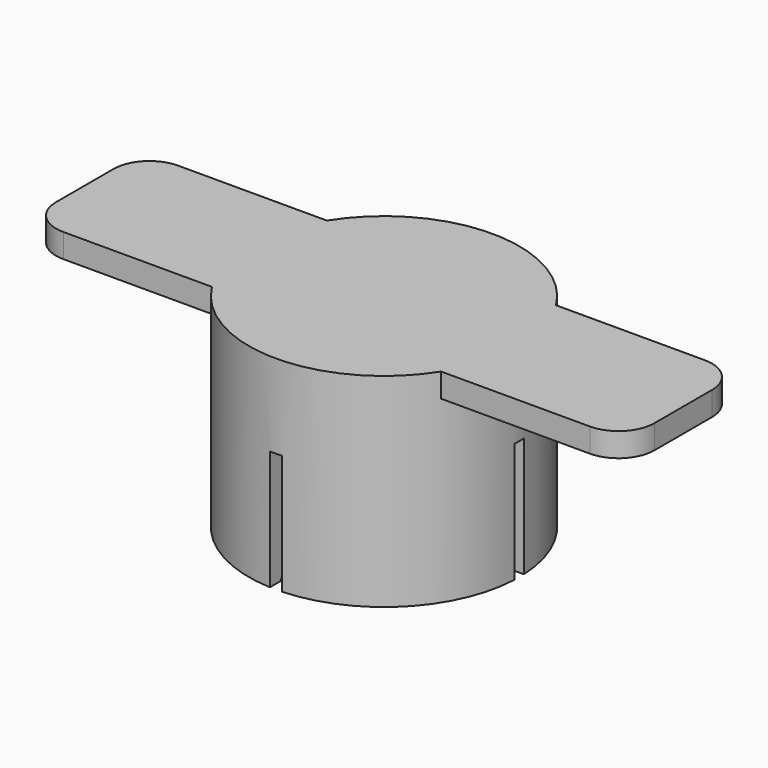
from build123d import *

# Parameters (mm, degrees)
F0_R         = 11.3
F0_R_2       = 9
F1_DEPTH     = 15
F2_R         = 11.3
F3_DEPTH     = 2
F5_START     = -5
F4_R         = 9.5
F4_R_2       = 7.1437360255
F5_DEPTH     = 3.1
F7_W         = 50
F7_H         = 12
F8_DEPTH     = 2
F9_R         = 3
F10_W        = 1
F10_H        = 12
F10_W_2      = 12
F10_H_2      = 1
F11_DEPTH    = 10
F12_SIZE     = 1.2
F13_T2_ANGLE = 179.6107254138
F13_T4_ANGLE = 179.6107254138
F13_T6_ANGLE = 179.6107254138
F13_T8_ANGLE = 179.6107254138


# Not quite as in the source:
# - a fillet or chamfer that OpenCascade refuses, or shapes differently, is made with other operations: its cross-section is extruded or revolved along the edge and cut away or added


with BuildPart() as f1:
    # F0 (on Top) → F1 (new body)
    with BuildSketch(Plane.XY):
        Circle(F0_R)
        Circle(F0_R_2, mode=Mode.SUBTRACT)
    extrude(amount=F1_DEPTH)

    # F2 (on face) → F3 (join)
    with BuildSketch(Plane.XY.offset(15)):
        Circle(F2_R)
    extrude(amount=F3_DEPTH)

    # F4 (on face) → F5 (cut)
    with BuildSketch(Plane(origin=(0, 0, 0), x_dir=(1, 0, 0), z_dir=(0, 0, -1)).offset(F5_START)):
        Circle(F4_R)
        Circle(F4_R_2, mode=Mode.SUBTRACT)
    extrude(amount=-F5_DEPTH, mode=Mode.SUBTRACT)

    # F6: fillet of radius 1.5 on 3 edges, made by hand

    # F6_s1 → F6_t2 (revolve)
    with BuildSketch(Plane.XZ):
        with BuildLine():
            ThreePointArc((9, 5), (9.3693063938, 5.5056615531), (9.5, 6.1180339887))
            Line((9.5, 6.1180339887), (9.53, 6.1180339887))
            Line((9.53, 6.1180339887), (9.53, 5))
            Line((9.53, 5), (9.5, 4.97))
            ThreePointArc((9.5, 4.97), (9.25, 4.97), (9.02, 4.9776393202))
            Line((9.02, 4.9776393202), (9, 5))
        make_face()
    revolve(axis=Axis((0, 0, 5), (0, 0, -1)))

    # F6_s3 → F6_t4 (revolve)
    with BuildSketch(Plane.XZ):
        with BuildLine():
            ThreePointArc((9.5, 6.9819660113), (9.3693063938, 7.5943384469), (9, 8.1))
            Line((9, 8.1), (9.02, 8.1223606798))
            ThreePointArc((9.02, 8.1223606798), (9.25, 8.13), (9.5, 8.13))
            Line((9.5, 8.13), (9.53, 8.1))
            Line((9.53, 8.1), (9.53, 6.9819660113))
            Line((9.53, 6.9819660113), (9.5, 6.9819660113))
        make_face()
    revolve(axis=Axis((0, 0, 8.1), (0, 0, -1)))

    # F7 (on face) → F8 (join)
    with BuildSketch(Plane.XY.offset(17)):
        Rectangle(F7_W, F7_H)
    extrude(amount=-F8_DEPTH)

    # F9
    f9_edges = [f1.edges().sort_by_distance(p)[0] for p in [
        (-25, 6, 16),
        (-25, -6, 16),
        (25, 6, 16),
        (25, -6, 16),
    ]]
    fillet(f9_edges, radius=F9_R)

    # F10 (on face) → F11 (cut)
    with BuildSketch(Plane(origin=(0, 0, 0), x_dir=(1, 0, 0), z_dir=(0, 0, -1))):
        with Locations((0, -6.5)):
            Rectangle(F10_W, F10_H)
        with Locations((-6.5, 0)):
            Rectangle(F10_W_2, F10_H_2)
        Rectangle(F10_W, F10_H_2)
        with Locations((6.5, 0)):
            Rectangle(F10_W_2, F10_H_2)
        with Locations((0, 6.5)):
            Rectangle(F10_W, F10_H)
    extrude(amount=-F11_DEPTH, mode=Mode.SUBTRACT)

    # F12
    f12_edges = [f1.edges().sort_by_distance(p)[0] for p in [
        (6.363961, 6.363961, 0),
        (-6.363961, 6.363961, 0),
        (-6.363961, -6.363961, 0),
        (6.363961, -6.363961, 0),
    ]]
    chamfer(f12_edges, length=F12_SIZE)

    # F13: fillet of radius 8 on 4 edges, made by hand

    # F13_s1 → F13_t2 (revolve, cut)
    with BuildSketch(Plane(origin=(0, 0, 0), x_dir=(0, 0, 1), z_dir=(0.7095047819, -0.7047006205, 0))):
        with BuildLine():
            ThreePointArc((0, -10.2), (2.0233712711, -9.3058463753), (4.2142615011, -9))
            Line((4.2142615011, -9), (1.2, -9))
            Line((1.2, -9), (0, -10.2))
        make_face()
    revolve(axis=Axis((0, 0, 1.2), (0, 0, 1)), revolution_arc=F13_T2_ANGLE, mode=Mode.SUBTRACT)

    # F13_s3 → F13_t4 (revolve, cut)
    with BuildSketch(Plane(origin=(0, 0, 0), x_dir=(0, 0, 1), z_dir=(0.7047006205, 0.7095047819, 0))):
        with BuildLine():
            ThreePointArc((0, -10.2), (2.0233712711, -9.3058463753), (4.2142615011, -9))
            Line((4.2142615011, -9), (1.2, -9))
            Line((1.2, -9), (0, -10.2))
        make_face()
    revolve(axis=Axis((0, 0, 1.2), (0, 0, 1)), revolution_arc=F13_T4_ANGLE, mode=Mode.SUBTRACT)

    # F13_s5 → F13_t6 (revolve, cut)
    with BuildSketch(Plane(origin=(0, 0, 0), x_dir=(0, 0, 1), z_dir=(-0.7047006205, -0.7095047819, 0))):
        with BuildLine():
            ThreePointArc((0, -10.2), (2.0233712711, -9.3058463753), (4.2142615011, -9))
            Line((4.2142615011, -9), (1.2, -9))
            Line((1.2, -9), (0, -10.2))
        make_face()
    revolve(axis=Axis((0, 0, 1.2), (0, 0, 1)), revolution_arc=F13_T6_ANGLE, mode=Mode.SUBTRACT)

    # F13_s7 → F13_t8 (revolve, cut)
    with BuildSketch(Plane(origin=(0, 0, 0), x_dir=(0, 0, 1), z_dir=(-0.7095047819, 0.7047006205, 0))):
        with BuildLine():
            ThreePointArc((0, -10.2), (2.0233712711, -9.3058463753), (4.2142615011, -9))
            Line((4.2142615011, -9), (1.2, -9))
            Line((1.2, -9), (0, -10.2))
        make_face()
    revolve(axis=Axis((0, 0, 1.2), (0, 0, 1)), revolution_arc=F13_T8_ANGLE, mode=Mode.SUBTRACT)


solid = f1.part
